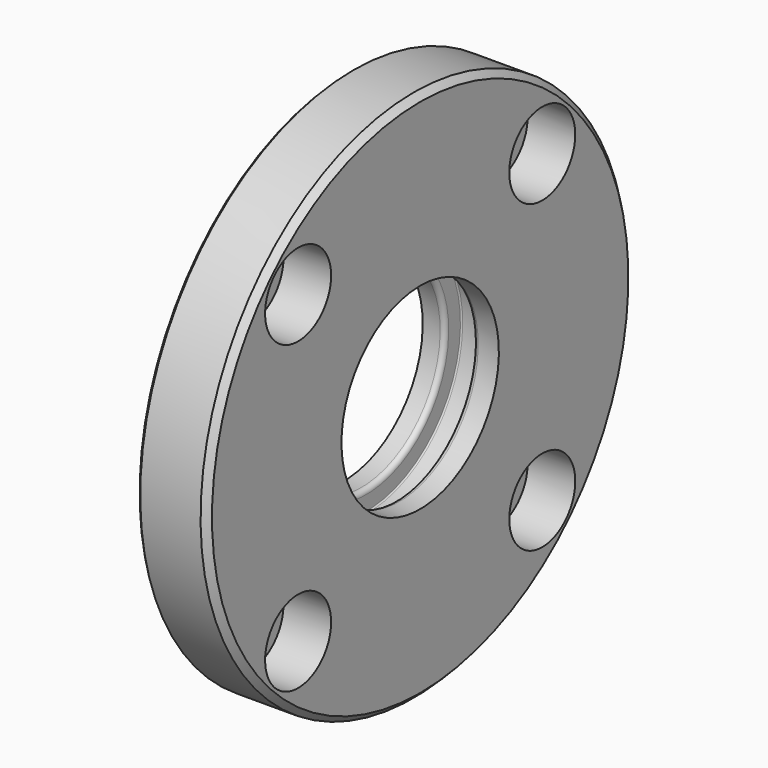
from build123d import *

# Parameters (mm, degrees)
F2_SIZE         = 1
F3_SIZE         = 0.5
F5_D            = 6.6
F5_CBORE_D      = 13
F5_CBORE_DEPTH  = 7.5
F5_COPIES_COUNT = 4


# Not quite as in the source:
# - a pattern or mirror of a feature is missing from the dataset's text; its kind, count and spacing are read off the source's solid


with BuildPart() as f1:
    # F0 (on Front) → F1 (revolve)
    with BuildSketch(Plane.XZ):
        with BuildLine():
            Line((-3.25, 15.5), (0, 15.5))
            Line((0, 15.5), (0, 42))
            Line((0, 42), (-11, 42))
            Line((-11, 42), (-11, 28))
            ThreePointArc((-11, 28), (-11.2928932188, 27.2928932188), (-12, 27))
            Line((-12, 27), (-13, 27))
            Line((-13, 27), (-13, 24))
            Line((-13, 24), (-12, 24))
            Line((-12, 24), (-12, 15.5))
            Line((-12, 15.5), (-9.25, 15.5))
            ThreePointArc((-9.25, 15.5), (-8.7196699141, 15.7196699141), (-8.5, 16.25))
            Line((-8.5, 16.25), (-8.5, 18.55))
            ThreePointArc((-8.5, 18.55), (-8.4414213562, 18.6914213562), (-8.3, 18.75))
            Line((-8.3, 18.75), (-4.2, 18.75))
            ThreePointArc((-4.2, 18.75), (-4.0585786438, 18.6914213562), (-4, 18.55))
            Line((-4, 18.55), (-4, 16.25))
            ThreePointArc((-4, 16.25), (-3.7803300859, 15.7196699141), (-3.25, 15.5))
        make_face()
    revolve(axis=Axis((-6.5, 0, 0), (-1, 0, 0)))

    # F2
    f2_edges = [f1.edges().sort_by_distance(p)[0] for p in [
        (0, 0, -42),
    ]]
    chamfer(f2_edges, length=F2_SIZE)

    # F3
    f3_edges = [f1.edges().sort_by_distance(p)[0] for p in [
        (-11, 0, -42),
    ]]
    chamfer(f3_edges, length=F3_SIZE)

    # F5 (through all)
    with Locations(Plane.YZ):
        with Locations((-24.0416305603, 24.0416305603)):
            f5 = CounterBoreHole(F5_D / 2, F5_CBORE_D / 2, F5_CBORE_DEPTH)

    # F5_copies: F5 ×4 about axis
    f5_copies_axis = Axis((0, 0, 0), (1, 0, 0))
    for i in range(1, F5_COPIES_COUNT):
        add(f5.rotate(f5_copies_axis, i * 360 / F5_COPIES_COUNT), mode=Mode.SUBTRACT)


solid = f1.part
